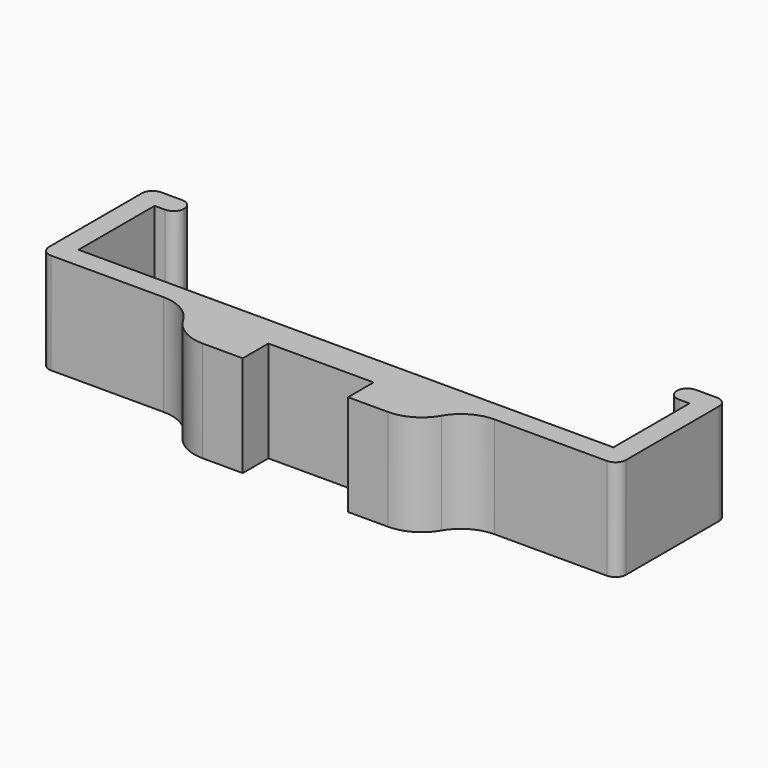
from build123d import *

# Parameters (mm, degrees)
F0_W     = 22
F0_H     = 5
F1_DEPTH = 12
F2_W     = 12.5
F2_H     = 3.8
F3_DEPTH = 12
F4_R     = 5
F5_R     = 1.24999


# Not quite as in the source:
# - a fillet or chamfer is up to 0.001 mm smaller than in the source, because OpenCascade refuses the exact size


with BuildPart() as f1:
    # F0 (on Top) → F1 (new body)
    with BuildSketch(Plane.XY):
        Polygon((31.75, -1.25), (31.75, 1.25), (-31.75, 1.25), (-31.75, -1.25), (-16, -1.25), (-11, -1.25), (11, -1.25), (16, -1.25), align=None)
        Polygon((31.75, 12.55), (31.75, 1.25), (31.75, -1.25), (34.25, -1.25), (34.25, 12.55), align=None)
        Polygon((-31.75, -1.25), (-31.75, 1.25), (-31.75, 12.55), (-34.25, 12.55), (-34.25, -1.25), align=None)
        Polygon((29.25, 12.55), (31.75, 12.55), (34.25, 12.55), (34.25, 15.05), (29.25, 15.05), align=None)
        Polygon((-34.25, 12.55), (-31.75, 12.55), (-29.25, 12.55), (-29.25, 15.05), (-34.25, 15.05), align=None)
        with BuildLine():
            ThreePointArc((11, -6.25), (14.5355339059, -4.7855339059), (16, -1.25))
            Line((16, -1.25), (11, -1.25))
            Line((11, -1.25), (11, -6.25))
        make_face()
        with BuildLine():
            Line((-11, -1.25), (-16, -1.25))
            ThreePointArc((-16, -1.25), (-14.5355339059, -4.7855339059), (-11, -6.25))
            Line((-11, -6.25), (-11, -1.25))
        make_face()
        with Locations((0, -3.75)):
            Rectangle(F0_W, F0_H)
    extrude(amount=F1_DEPTH)

    # F2 (on face) → F3 (cut, through all)
    with BuildSketch(Plane.XY.offset(12)):
        with Locations((0, -4.35)):
            Rectangle(F2_W, F2_H)
    extrude(amount=-F3_DEPTH, mode=Mode.SUBTRACT)

    # F4
    f4_edges = [f1.edges().sort_by_distance(p)[0] for p in [
        (16, -1.25, 6),
        (-16, -1.25, 6),
    ]]
    fillet(f4_edges, radius=F4_R)

    # F5 (radius 1.25 in the source; OpenCascade refuses exactly that, so slightly less here)
    f5_edges = [f1.edges().sort_by_distance(p)[0] for p in [
        (-34.25, -1.25, 6),
        (34.25, -1.25, 6),
        (-34.25, 15.05, 6),
        (-29.25, 15.05, 6),
        (-29.25, 12.55, 6),
        (29.25, 12.55, 6),
        (29.25, 15.05, 6),
        (34.25, 15.05, 6),
    ]]
    fillet(f5_edges, radius=F5_R)


solid = f1.part
